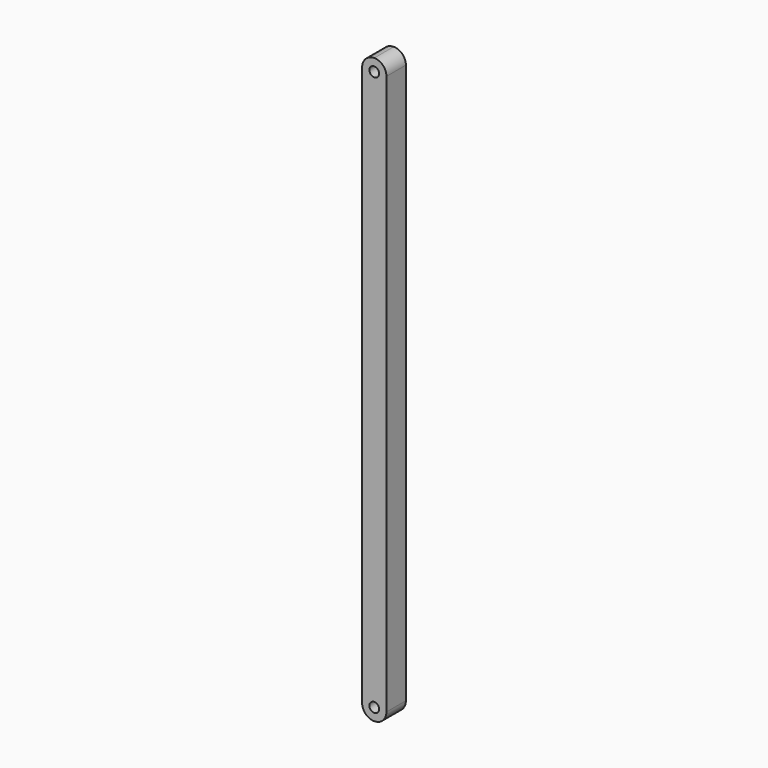
from build123d import *

# Parameters (mm, degrees)
F0_W     = 25
F0_H     = 600
F1_DEPTH = 25
F2_R     = 12.49999
F3_R     = 12.49999
F4_R     = 5
F5_DEPTH = 25


# Not quite as in the source:
# - a fillet or chamfer is up to 0.001 mm smaller than in the source, because OpenCascade refuses the exact size
# - a pattern or mirror of a feature is missing from the dataset's text; its kind, count and spacing are read off the source's solid


with BuildPart() as f1:
    # F0 (on Front) → F1 (new body)
    with BuildSketch(Plane.XZ):
        Rectangle(F0_W, F0_H)
    extrude(amount=F1_DEPTH)

    # F2 (radius 12.5 in the source; OpenCascade refuses exactly that, so slightly less here)
    f2_edges = [f1.edges().sort_by_distance(p)[0] for p in [
        (-12.5, -12.5, 300),
        (12.5, -12.5, 300),
    ]]
    fillet(f2_edges, radius=F2_R)

    # F3 (radius 12.5 in the source; OpenCascade refuses exactly that, so slightly less here)
    f3_edges = [f1.edges().sort_by_distance(p)[0] for p in [
        (-12.5, -12.5, -300),
        (12.5, -12.5, -300),
    ]]
    fillet(f3_edges, radius=F3_R)

    # F4 (on face) → F5 (cut)
    with BuildSketch(Plane.XZ.offset(25)):
        with Locations((0, 287.5)):
            Circle(F4_R)
    f5 = extrude(amount=-F5_DEPTH, mode=Mode.SUBTRACT)

    # F5_copies: F5 across plane
    add(f5.mirror(Plane(origin=(0, 0, 0), x_dir=(-1, 0, 0), z_dir=(0, 0, -1))), mode=Mode.SUBTRACT)


solid = f1.part
